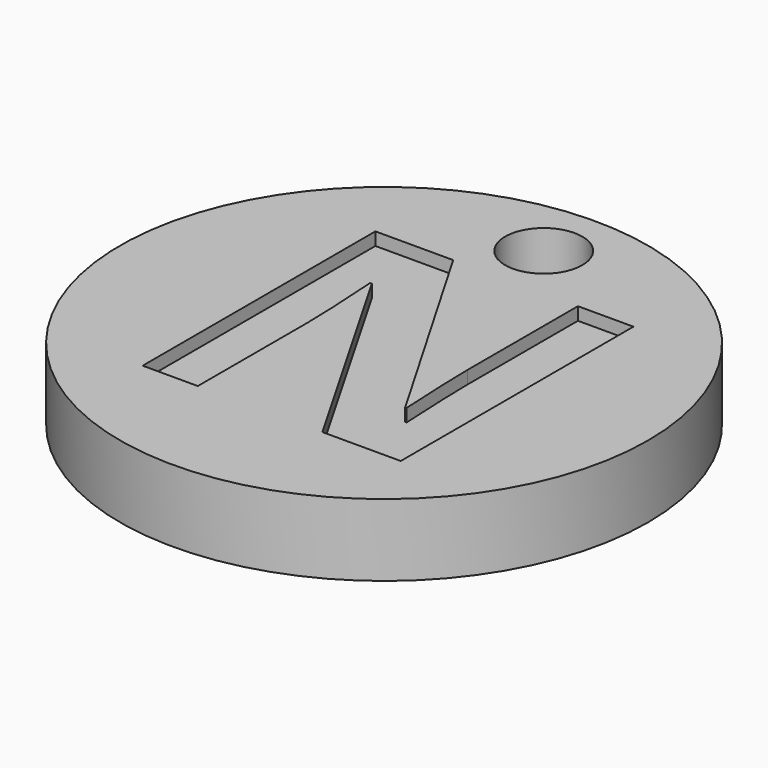
from build123d import *

# Parameters (mm, degrees)
F0_R         = 10.25
F1_DEPTH     = 2.8
F2_TEXT_SIZE = 15.8236071002
F3_DEPTH     = 0.5
F4_R         = 1.5
F5_DEPTH     = 25


# Not quite as in the source:
# - Text() gives the source's letters only with a copy of the font that has no kerning and outlines rounded to 1/6400 em; it was checked with that copy


with BuildPart() as f1:
    # F0 (on Top) → F1 (new body)
    with BuildSketch(Plane.XY):
        Circle(F0_R)
    extrude(amount=F1_DEPTH)

    # F2 (on face) → F3 (cut)
    with BuildSketch(Plane.XY.offset(2.8)):
        with Locations((-6.208152945, -5.7354117744)):
            Text('N', F2_TEXT_SIZE, font='Open Sans', font_style=FontStyle.BOLD, text_align=(TextAlign.LEFT, TextAlign.BOTTOM))
    extrude(amount=-F3_DEPTH, mode=Mode.SUBTRACT)

    # F4 (on face) → F5 (cut)
    with BuildSketch(Plane.XY.offset(2.8)):
        with Locations((0, 7.75)):
            Circle(F4_R)
    extrude(amount=-F5_DEPTH, mode=Mode.SUBTRACT)


solid = f1.part
